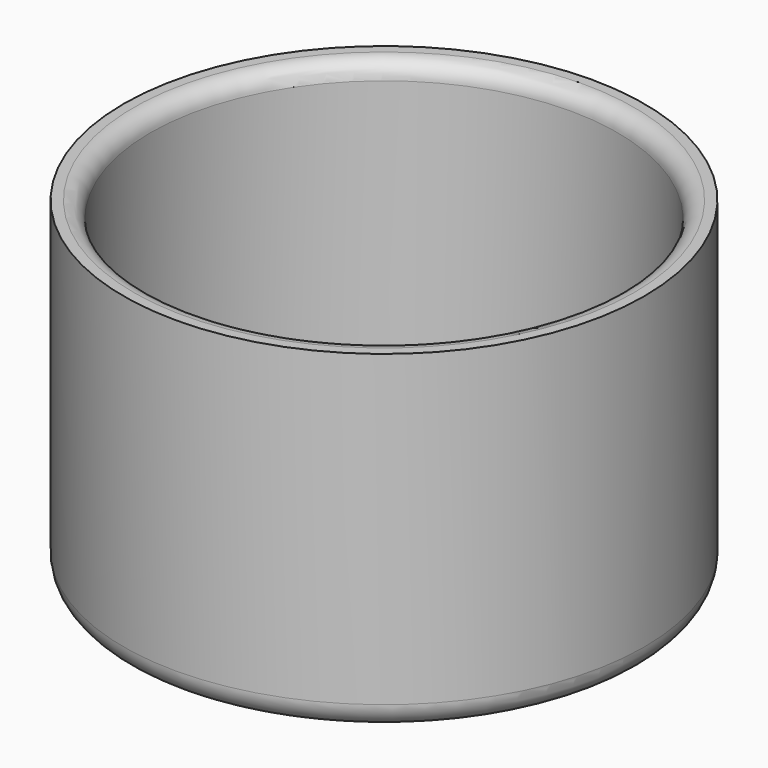
from build123d import *

# Parameters (mm, degrees)
F0_R        = 15.6
F0_R_2      = 14
F0_R_3      = 2
F1_DEPTH    = 3
F2_DEPTH    = 20
F3_R        = 1.5
F4_R        = 1
F5_R        = 2
F6_DEPTH    = 3
F7_T1_DEPTH = 3


# Not quite as in the source:
# - a fillet or chamfer that OpenCascade refuses, or shapes differently, is made with other operations: its cross-section is extruded or revolved along the edge and cut away or added


with BuildPart() as f1:
    # F0 (on Top) → F1 (new body)
    with BuildSketch(Plane.XY):
        Circle(F0_R)
        Circle(F0_R_2, mode=Mode.SUBTRACT)
        Circle(F0_R_2)
        Circle(F0_R_3, mode=Mode.SUBTRACT)
        Circle(F0_R_3)
    extrude(amount=F1_DEPTH)

    # F0 (on Top) → F2 (join)
    with BuildSketch(Plane.XY):
        Circle(F0_R)
        Circle(F0_R_2, mode=Mode.SUBTRACT)
    extrude(amount=F2_DEPTH)

    # F3
    f3_edges = [f1.edges().sort_by_distance(p)[0] for p in [
        (-15.6, 0, 0),
    ]]
    fillet(f3_edges, radius=F3_R)

    # F4
    f4_edges = [f1.edges().sort_by_distance(p)[0] for p in [
        (-14, 0, 20),
    ]]
    fillet(f4_edges, radius=F4_R)

    # F5 (on face) + F0 (on Top) → F6 (cut, through all)
    with BuildSketch(Plane.XY):
        with BuildLine():
            add(Edge.make_bspline(
                [(0, -2.5137708586), (0, -4.1458795261), (-1.7837920859, -8.9341028845), (-10.8913647651, -3.867257191), (-4.0863468312, 3.7691965699), (0, 8.5115667947)],
                knots=[0, 0, 0, 0, 0.2681845993, 0.5480579368, 1, 1, 1, 1], degree=3))
            add(Edge.make_bspline(
                [(0, -2.5137708586), (0, -4.1458795261), (1.7837920859, -8.9341028845), (10.8913647651, -3.867257191), (4.0863468312, 3.7691965699), (0, 8.5115667947)],
                knots=[0, 0, 0, 0, 0.2681845993, 0.5480579368, 1, 1, 1, 1], degree=3))
        make_face()
        Circle(F5_R, mode=Mode.SUBTRACT)
    with BuildSketch(Plane.XY):
        Circle(F0_R_3)
    extrude(amount=F6_DEPTH, mode=Mode.SUBTRACT)

    # F7: fillet of radius 0.4 on 1 edges, made by hand

    # F7_s2 → F7_t1 (cut)
    with BuildSketch(Plane.XY):
        with BuildLine():
            ThreePointArc((0.3762881855, -4.5548185088), (0, -4.2904916507), (-0.3762881855, -4.5548185088))
            Line((-0.3762881855, -4.5548185088), (-0.3838139492, -4.5521050459))
            ThreePointArc((-0.3838139492, -4.5521050459), (-0.1103093457, -3.5489845707), (-0.008, -2.5137708586))
            Line((-0.008, -2.5137708586), (0.008, -2.5137708586))
            ThreePointArc((0.008, -2.5137708586), (0.1103093457, -3.5489845707), (0.3838139492, -4.5521050459))
            Line((0.3838139492, -4.5521050459), (0.3762881855, -4.5548185088))
        make_face()
    extrude(amount=F7_T1_DEPTH, mode=Mode.SUBTRACT)


solid = f1.part
